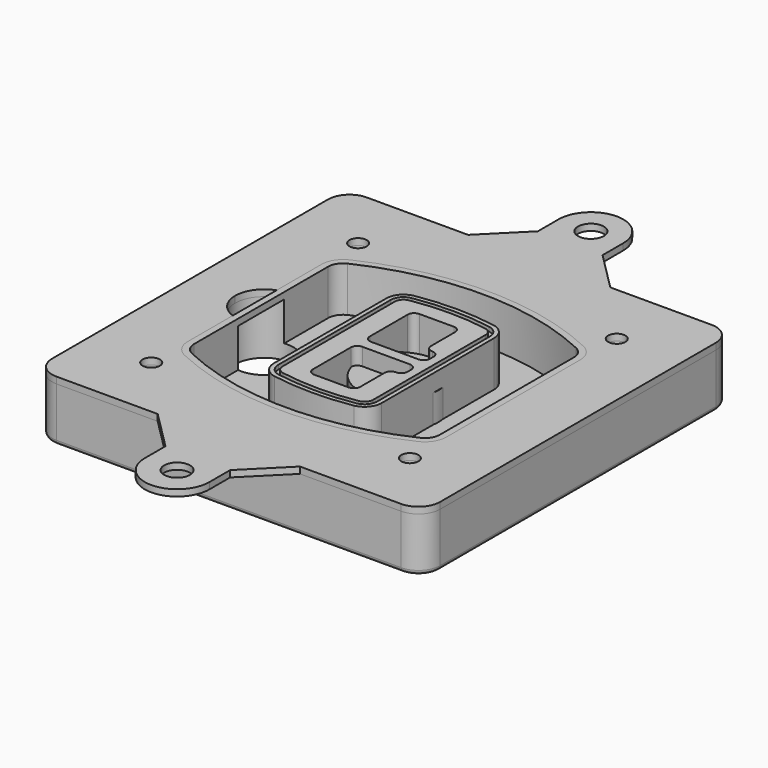
from build123d import *

# Parameters (mm, degrees)
F0_R      = 4
F1_DEPTH  = 25
F2_DEPTH  = 3
F3_DEPTH  = 18
F5_DEPTH  = 21
F6_DEPTH  = 2
F8_DEPTH  = 20
F9_DEPTH  = 16
F10_DEPTH = 25
F7_R      = 6
F7_R_2    = 4
F11_DEPTH = 6
F13_DEPTH = 9
F15_R     = 2
F16_R     = 6
F16_R_2   = 4
F17_DEPTH = 3


# Not quite as in the source:
# - a feature of the source that left no trace in its solid (it failed there, or was rolled back) is left out
# - a feature names something its author has since deleted; it is built from what else it names


with BuildPart() as f1:
    # F0 (on Top) → F1 (new body)
    with BuildSketch(Plane.XY):
        with BuildLine():
            ThreePointArc((-90, -80), (-87.0710678119, -87.0710678119), (-80, -90))
            Line((-80, -90), (80, -90))
            ThreePointArc((80, -90), (87.0710678119, -87.0710678119), (90, -80))
            Line((90, -80), (90, 80))
            ThreePointArc((90, 80), (87.0710678119, 87.0710678119), (80, 90))
            Line((80, 90), (-80, 90))
            ThreePointArc((-80, 90), (-87.0710678119, 87.0710678119), (-90, 80))
            Line((-90, 80), (-90, -80))
        make_face()
        with Locations((-60, -60)):
            Circle(F0_R, mode=Mode.SUBTRACT)
        with Locations((60, -60)):
            Circle(F0_R, mode=Mode.SUBTRACT)
        with Locations((-60, 60)):
            Circle(F0_R, mode=Mode.SUBTRACT)
        with BuildLine():
            ThreePointArc((-64, 38.8308515907), (-61.8195654598, 46.3340424013), (-55.9574468085, 51.5000594398))
            ThreePointArc((-55.9574468085, 51.5000594398), (0, 64), (55.9574468085, 51.5000594398))
            ThreePointArc((55.9574468085, 51.5000594398), (61.8195654598, 46.3340424013), (64, 38.8308515907))
            Line((64, 38.8308515907), (64, -38.8308515907))
            ThreePointArc((64, -38.8308515907), (61.8195654598, -46.3340424013), (55.9574468085, -51.5000594398))
            ThreePointArc((55.9574468085, -51.5000594398), (0, -64), (-55.9574468085, -51.5000594398))
            ThreePointArc((-55.9574468085, -51.5000594398), (-61.8195654598, -46.3340424013), (-64, -38.8308515907))
            Line((-64, -38.8308515907), (-64, 38.8308515907))
        make_face(mode=Mode.SUBTRACT)
        with Locations((60, 60)):
            Circle(F0_R, mode=Mode.SUBTRACT)
        with BuildLine():
            ThreePointArc((55.9574468085, 51.5000594398), (0, 64), (-55.9574468085, 51.5000594398))
            ThreePointArc((-55.9574468085, 51.5000594398), (-61.8195654598, 46.3340424013), (-64, 38.8308515907))
            Line((-64, 38.8308515907), (-64, -38.8308515907))
            ThreePointArc((-64, -38.8308515907), (-61.8195654598, -46.3340424013), (-55.9574468085, -51.5000594398))
            ThreePointArc((-55.9574468085, -51.5000594398), (0, -64), (55.9574468085, -51.5000594398))
            ThreePointArc((55.9574468085, -51.5000594398), (61.8195654598, -46.3340424013), (64, -38.8308515907))
            Line((64, -38.8308515907), (64, 38.8308515907))
            ThreePointArc((64, 38.8308515907), (61.8195654598, 46.3340424013), (55.9574468085, 51.5000594398))
        make_face()
        with BuildLine():
            Line((-60, -38.8308515907), (-60, 38.8308515907))
            ThreePointArc((-60, 38.8308515907), (-58.442546757, 44.1902735983), (-54.2553191489, 47.8802857686))
            ThreePointArc((-54.2553191489, 47.8802857686), (0, 60), (54.2553191489, 47.8802857686))
            ThreePointArc((54.2553191489, 47.8802857686), (58.442546757, 44.1902735983), (60, 38.8308515907))
            Line((60, 38.8308515907), (60, -38.8308515907))
            ThreePointArc((60, -38.8308515907), (58.442546757, -44.1902735983), (54.2553191489, -47.8802857686))
            ThreePointArc((54.2553191489, -47.8802857686), (0, -60), (-54.2553191489, -47.8802857686))
            ThreePointArc((-54.2553191489, -47.8802857686), (-58.442546757, -44.1902735983), (-60, -38.8308515907))
        make_face(mode=Mode.SUBTRACT)
        with BuildLine():
            ThreePointArc((-54.2553191489, 47.8802857686), (-58.442546757, 44.1902735983), (-60, 38.8308515907))
            Line((-60, 38.8308515907), (-60, -38.8308515907))
            ThreePointArc((-60, -38.8308515907), (-58.442546757, -44.1902735983), (-54.2553191489, -47.8802857686))
            ThreePointArc((-54.2553191489, -47.8802857686), (0, -60), (54.2553191489, -47.8802857686))
            ThreePointArc((54.2553191489, -47.8802857686), (58.442546757, -44.1902735983), (60, -38.8308515907))
            Line((60, -38.8308515907), (60, 38.8308515907))
            ThreePointArc((60, 38.8308515907), (58.442546757, 44.1902735983), (54.2553191489, 47.8802857686))
            ThreePointArc((54.2553191489, 47.8802857686), (0, 60), (-54.2553191489, 47.8802857686))
        make_face()
        with BuildLine():
            ThreePointArc((52.9787234043, 45.1654555152), (55.9097827299, 42.582446996), (57, 38.8308515907))
            Line((57, 38.8308515907), (57, -38.8308515907))
            ThreePointArc((57, -38.8308515907), (55.9097827299, -42.582446996), (52.9787234043, -45.1654555152))
            ThreePointArc((52.9787234043, -45.1654555152), (0, -57), (-52.9787234043, -45.1654555152))
            ThreePointArc((-52.9787234043, -45.1654555152), (-55.9097827299, -42.582446996), (-57, -38.8308515907))
            Line((-57, -38.8308515907), (-57, 38.8308515907))
            ThreePointArc((-57, 38.8308515907), (-55.9097827299, 42.582446996), (-52.9787234043, 45.1654555152))
            ThreePointArc((-52.9787234043, 45.1654555152), (0, 57), (52.9787234043, 45.1654555152))
        make_face(mode=Mode.SUBTRACT)
        with BuildLine():
            Line((57, -38.8308515907), (57, 38.8308515907))
            ThreePointArc((57, 38.8308515907), (55.9097827299, 42.582446996), (52.9787234043, 45.1654555152))
            ThreePointArc((52.9787234043, 45.1654555152), (0, 57), (-52.9787234043, 45.1654555152))
            ThreePointArc((-52.9787234043, 45.1654555152), (-55.9097827299, 42.582446996), (-57, 38.8308515907))
            Line((-57, 38.8308515907), (-57, -38.8308515907))
            ThreePointArc((-57, -38.8308515907), (-55.9097827299, -42.582446996), (-52.9787234043, -45.1654555152))
            ThreePointArc((-52.9787234043, -45.1654555152), (0, -57), (52.9787234043, -45.1654555152))
            ThreePointArc((52.9787234043, -45.1654555152), (55.9097827299, -42.582446996), (57, -38.8308515907))
        make_face()
    extrude(amount=-F1_DEPTH)

    # F0 (on Top) → F2 (join)
    with BuildSketch(Plane.XY):
        with BuildLine():
            ThreePointArc((-54.2553191489, 47.8802857686), (-58.442546757, 44.1902735983), (-60, 38.8308515907))
            Line((-60, 38.8308515907), (-60, -38.8308515907))
            ThreePointArc((-60, -38.8308515907), (-58.442546757, -44.1902735983), (-54.2553191489, -47.8802857686))
            ThreePointArc((-54.2553191489, -47.8802857686), (0, -60), (54.2553191489, -47.8802857686))
            ThreePointArc((54.2553191489, -47.8802857686), (58.442546757, -44.1902735983), (60, -38.8308515907))
            Line((60, -38.8308515907), (60, 38.8308515907))
            ThreePointArc((60, 38.8308515907), (58.442546757, 44.1902735983), (54.2553191489, 47.8802857686))
            ThreePointArc((54.2553191489, 47.8802857686), (0, 60), (-54.2553191489, 47.8802857686))
        make_face()
        with BuildLine():
            ThreePointArc((52.9787234043, 45.1654555152), (55.9097827299, 42.582446996), (57, 38.8308515907))
            Line((57, 38.8308515907), (57, -38.8308515907))
            ThreePointArc((57, -38.8308515907), (55.9097827299, -42.582446996), (52.9787234043, -45.1654555152))
            ThreePointArc((52.9787234043, -45.1654555152), (0, -57), (-52.9787234043, -45.1654555152))
            ThreePointArc((-52.9787234043, -45.1654555152), (-55.9097827299, -42.582446996), (-57, -38.8308515907))
            Line((-57, -38.8308515907), (-57, 38.8308515907))
            ThreePointArc((-57, 38.8308515907), (-55.9097827299, 42.582446996), (-52.9787234043, 45.1654555152))
            ThreePointArc((-52.9787234043, 45.1654555152), (0, 57), (52.9787234043, 45.1654555152))
        make_face(mode=Mode.SUBTRACT)
    extrude(amount=F2_DEPTH)

    # F0 (on Top) → F3 (cut)
    with BuildSketch(Plane.XY):
        with BuildLine():
            Line((57, -38.8308515907), (57, 38.8308515907))
            ThreePointArc((57, 38.8308515907), (55.9097827299, 42.582446996), (52.9787234043, 45.1654555152))
            ThreePointArc((52.9787234043, 45.1654555152), (0, 57), (-52.9787234043, 45.1654555152))
            ThreePointArc((-52.9787234043, 45.1654555152), (-55.9097827299, 42.582446996), (-57, 38.8308515907))
            Line((-57, 38.8308515907), (-57, -38.8308515907))
            ThreePointArc((-57, -38.8308515907), (-55.9097827299, -42.582446996), (-52.9787234043, -45.1654555152))
            ThreePointArc((-52.9787234043, -45.1654555152), (0, -57), (52.9787234043, -45.1654555152))
            ThreePointArc((52.9787234043, -45.1654555152), (55.9097827299, -42.582446996), (57, -38.8308515907))
        make_face()
    extrude(amount=-F3_DEPTH, mode=Mode.SUBTRACT)

    # F4 (on face) → F5 (join, through all)
    with BuildSketch(Plane.XY.offset(3)):
        with BuildLine():
            ThreePointArc((-25, -32.5662280692), (-23.1122504785, -37.7276614059), (-18.3399014778, -40.4532214146))
            ThreePointArc((-18.3399014778, -40.4532214146), (0, -42), (18.3399014778, -40.4532214146))
            ThreePointArc((18.3399014778, -40.4532214146), (23.1122504785, -37.7276614059), (25, -32.5662280692))
            Line((25, -32.5662280692), (25, 32.5662280692))
            ThreePointArc((25, 32.5662280692), (23.1122504785, 37.7276614059), (18.3399014778, 40.4532214146))
            ThreePointArc((18.3399014778, 40.4532214146), (0, 42), (-18.3399014778, 40.4532214146))
            ThreePointArc((-18.3399014778, 40.4532214146), (-23.1122504785, 37.7276614059), (-25, 32.5662280692))
            Line((-25, 32.5662280692), (-25, -32.5662280692))
        make_face()
        with BuildLine():
            ThreePointArc((18.0049261084, 38.4814730782), (21.5841878588, 36.4373030717), (23, 32.5662280692))
            Line((23, 32.5662280692), (23, -32.5662280692))
            ThreePointArc((23, -32.5662280692), (21.5841878588, -36.4373030717), (18.0049261084, -38.4814730782))
            ThreePointArc((18.0049261084, -38.4814730782), (0, -40), (-18.0049261084, -38.4814730782))
            ThreePointArc((-18.0049261084, -38.4814730782), (-21.5841878588, -36.4373030717), (-23, -32.5662280692))
            Line((-23, -32.5662280692), (-23, 32.5662280692))
            ThreePointArc((-23, 32.5662280692), (-21.5841878588, 36.4373030717), (-18.0049261084, 38.4814730782))
            ThreePointArc((-18.0049261084, 38.4814730782), (0, 40), (18.0049261084, 38.4814730782))
        make_face(mode=Mode.SUBTRACT)
        with BuildLine():
            Line((23, -32.5662280692), (23, 32.5662280692))
            ThreePointArc((23, 32.5662280692), (21.5841878588, 36.4373030717), (18.0049261084, 38.4814730782))
            ThreePointArc((18.0049261084, 38.4814730782), (0, 40), (-18.0049261084, 38.4814730782))
            ThreePointArc((-18.0049261084, 38.4814730782), (-21.5841878588, 36.4373030717), (-23, 32.5662280692))
            Line((-23, 32.5662280692), (-23, -32.5662280692))
            ThreePointArc((-23, -32.5662280692), (-21.5841878588, -36.4373030717), (-18.0049261084, -38.4814730782))
            ThreePointArc((-18.0049261084, -38.4814730782), (0, -40), (18.0049261084, -38.4814730782))
            ThreePointArc((18.0049261084, -38.4814730782), (21.5841878588, -36.4373030717), (23, -32.5662280692))
        make_face()
        with BuildLine():
            ThreePointArc((17.6699507389, 36.5097247419), (20.0561252392, 35.1469447375), (21, 32.5662280692))
            Line((21, 32.5662280692), (21, -32.5662280692))
            ThreePointArc((21, -32.5662280692), (20.0561252392, -35.1469447375), (17.6699507389, -36.5097247419))
            ThreePointArc((17.6699507389, -36.5097247419), (0, -38), (-17.6699507389, -36.5097247419))
            ThreePointArc((-17.6699507389, -36.5097247419), (-20.0561252392, -35.1469447375), (-21, -32.5662280692))
            Line((-21, -32.5662280692), (-21, 32.5662280692))
            ThreePointArc((-21, 32.5662280692), (-20.0561252392, 35.1469447375), (-17.6699507389, 36.5097247419))
            ThreePointArc((-17.6699507389, 36.5097247419), (0, 38), (17.6699507389, 36.5097247419))
        make_face(mode=Mode.SUBTRACT)
        with BuildLine():
            Line((21, -32.5662280692), (21, 32.5662280692))
            ThreePointArc((21, 32.5662280692), (20.0561252392, 35.1469447375), (17.6699507389, 36.5097247419))
            ThreePointArc((17.6699507389, 36.5097247419), (0, 38), (-17.6699507389, 36.5097247419))
            ThreePointArc((-17.6699507389, 36.5097247419), (-20.0561252392, 35.1469447375), (-21, 32.5662280692))
            Line((-21, 32.5662280692), (-21, -32.5662280692))
            ThreePointArc((-21, -32.5662280692), (-20.0561252392, -35.1469447375), (-17.6699507389, -36.5097247419))
            ThreePointArc((-17.6699507389, -36.5097247419), (0, -38), (17.6699507389, -36.5097247419))
            ThreePointArc((17.6699507389, -36.5097247419), (20.0561252392, -35.1469447375), (21, -32.5662280692))
        make_face()
        with BuildLine():
            Line((-8, -2.5), (14, -2.5))
            ThreePointArc((14, -2.5), (16.1213203436, -3.3786796564), (17, -5.5))
            Line((17, -5.5), (17, -7.5))
            ThreePointArc((17, -7.5), (16.1213203436, -9.6213203436), (14, -10.5))
            ThreePointArc((14, -10.5), (11.8786796564, -11.3786796564), (11, -13.5))
            Line((11, -13.5), (11, -27.5))
            ThreePointArc((11, -27.5), (10.1213203436, -29.6213203436), (8, -30.5))
            Line((8, -30.5), (-8, -30.5))
            ThreePointArc((-8, -30.5), (-10.1213203436, -29.6213203436), (-11, -27.5))
            Line((-11, -27.5), (-11, -5.5))
            ThreePointArc((-11, -5.5), (-10.1213203436, -3.3786796564), (-8, -2.5))
        make_face(mode=Mode.SUBTRACT)
        with BuildLine():
            ThreePointArc((-8, 2.5), (-10.1213203436, 3.3786796564), (-11, 5.5))
            Line((-11, 5.5), (-11, 27.5))
            ThreePointArc((-11, 27.5), (-10.1213203436, 29.6213203436), (-8, 30.5))
            Line((-8, 30.5), (8, 30.5))
            ThreePointArc((8, 30.5), (10.1213203436, 29.6213203436), (11, 27.5))
            Line((11, 27.5), (11, 13.5))
            ThreePointArc((11, 13.5), (11.8786796564, 11.3786796564), (14, 10.5))
            ThreePointArc((14, 10.5), (16.1213203436, 9.6213203436), (17, 7.5))
            Line((17, 7.5), (17, 5.5))
            ThreePointArc((17, 5.5), (16.1213203436, 3.3786796564), (14, 2.5))
            Line((14, 2.5), (-8, 2.5))
        make_face(mode=Mode.SUBTRACT)
    extrude(amount=-F5_DEPTH)

    # F4 (on face) → F6 (cut)
    with BuildSketch(Plane.XY.offset(3)):
        with BuildLine():
            Line((23, -32.5662280692), (23, 32.5662280692))
            ThreePointArc((23, 32.5662280692), (21.5841878588, 36.4373030717), (18.0049261084, 38.4814730782))
            ThreePointArc((18.0049261084, 38.4814730782), (0, 40), (-18.0049261084, 38.4814730782))
            ThreePointArc((-18.0049261084, 38.4814730782), (-21.5841878588, 36.4373030717), (-23, 32.5662280692))
            Line((-23, 32.5662280692), (-23, -32.5662280692))
            ThreePointArc((-23, -32.5662280692), (-21.5841878588, -36.4373030717), (-18.0049261084, -38.4814730782))
            ThreePointArc((-18.0049261084, -38.4814730782), (0, -40), (18.0049261084, -38.4814730782))
            ThreePointArc((18.0049261084, -38.4814730782), (21.5841878588, -36.4373030717), (23, -32.5662280692))
        make_face()
        with BuildLine():
            ThreePointArc((17.6699507389, 36.5097247419), (20.0561252392, 35.1469447375), (21, 32.5662280692))
            Line((21, 32.5662280692), (21, -32.5662280692))
            ThreePointArc((21, -32.5662280692), (20.0561252392, -35.1469447375), (17.6699507389, -36.5097247419))
            ThreePointArc((17.6699507389, -36.5097247419), (0, -38), (-17.6699507389, -36.5097247419))
            ThreePointArc((-17.6699507389, -36.5097247419), (-20.0561252392, -35.1469447375), (-21, -32.5662280692))
            Line((-21, -32.5662280692), (-21, 32.5662280692))
            ThreePointArc((-21, 32.5662280692), (-20.0561252392, 35.1469447375), (-17.6699507389, 36.5097247419))
            ThreePointArc((-17.6699507389, 36.5097247419), (0, 38), (17.6699507389, 36.5097247419))
        make_face(mode=Mode.SUBTRACT)
    extrude(amount=-F6_DEPTH, mode=Mode.SUBTRACT)

    # F7 (on face) → F8 (join)
    with BuildSketch(Plane(origin=(0, 0, -25), x_dir=(1, 0, 0), z_dir=(0, 0, -1))):
        with BuildLine():
            ThreePointArc((-6.71157564, 0), (6.7567035675, 13.4682792075), (20.224982775, 0))
            Line((20.224982775, 0), (25.224982775, 0))
            ThreePointArc((25.224982775, 0), (6.7567035675, 18.4682792075), (-11.71157564, 0))
            Line((-11.71157564, 0), (-6.71157564, 0))
        make_face()
        with BuildLine():
            Line((-6.71157564, 0), (20.224982775, 0))
            ThreePointArc((20.224982775, 0), (6.7567035675, 13.4682792075), (-6.71157564, 0))
        make_face()
        with BuildLine():
            ThreePointArc((-6.71157564, 0), (6.7567035675, -13.4682792075), (20.224982775, 0))
            Line((20.224982775, 0), (-6.71157564, 0))
        make_face()
        with BuildLine():
            Line((25.224982775, 0), (20.224982775, 0))
            ThreePointArc((20.224982775, 0), (6.7567035675, -13.4682792075), (-6.71157564, 0))
            Line((-6.71157564, 0), (-11.71157564, 0))
            ThreePointArc((-11.71157564, 0), (6.7567035675, -18.4682792075), (25.224982775, 0))
        make_face()
    extrude(amount=-F8_DEPTH)

    # F7 (on face) → F9 (cut)
    with BuildSketch(Plane(origin=(0, 0, -25), x_dir=(1, 0, 0), z_dir=(0, 0, -1))):
        with BuildLine():
            Line((-6.71157564, 0), (20.224982775, 0))
            ThreePointArc((20.224982775, 0), (6.7567035675, 13.4682792075), (-6.71157564, 0))
        make_face()
        with BuildLine():
            ThreePointArc((-6.71157564, 0), (6.7567035675, -13.4682792075), (20.224982775, 0))
            Line((20.224982775, 0), (-6.71157564, 0))
        make_face()
    extrude(amount=-F9_DEPTH, mode=Mode.SUBTRACT)

    # F7 (on face) → F10 (cut)
    with BuildSketch(Plane(origin=(0, 0, -25), x_dir=(1, 0, 0), z_dir=(0, 0, -1))):
        with BuildLine():
            Line((-69.0318229325, 0), (-42.0952645175, 0))
            ThreePointArc((-42.0952645175, 0), (-55.563543725, 13.4682792075), (-69.0318229325, 0))
        make_face()
        with BuildLine():
            ThreePointArc((-69.0318229325, 0), (-55.563543725, -13.4682792075), (-42.0952645175, 0))
            Line((-42.0952645175, 0), (-69.0318229325, 0))
        make_face()
    extrude(amount=-F10_DEPTH, mode=Mode.SUBTRACT)

    # F7 (on face) → F11 (cut)
    with BuildSketch(Plane(origin=(0, 0, -25), x_dir=(1, 0, 0), z_dir=(0, 0, -1))):
        with Locations((60, -60)):
            Circle(F7_R)
        with Locations((60, -60)):
            Circle(F7_R_2, mode=Mode.SUBTRACT)
        with Locations((-60, -60)):
            Circle(F7_R)
        with Locations((-60, -60)):
            Circle(F7_R_2, mode=Mode.SUBTRACT)
        with Locations((-60, 60)):
            Circle(F7_R)
        with Locations((-60, 60)):
            Circle(F7_R_2, mode=Mode.SUBTRACT)
        with Locations((60, 60)):
            Circle(F7_R)
        with Locations((60, 60)):
            Circle(F7_R_2, mode=Mode.SUBTRACT)
    extrude(amount=-F11_DEPTH, mode=Mode.SUBTRACT)

    # F12 (on face) → F13 (cut, through all)
    with BuildSketch(Plane(origin=(0, 0, -9), x_dir=(1, 0, 0), z_dir=(0, 0, -1))):
        with BuildLine():
            ThreePointArc((20.224982775, 0), (20.1663399806, 1.2554664788), (19.9909222755, 2.5))
            Line((19.9909222755, 2.5), (14, 2.5))
            ThreePointArc((14, 2.5), (16.1213203436, 3.3786796564), (17, 5.5))
            Line((17, 5.5), (17, 7.5))
            ThreePointArc((17, 7.5), (16.1213203436, 9.6213203436), (14, 10.5))
            ThreePointArc((14, 10.5), (12.1627255951, 11.1284134507), (11.0951631559, 12.750384826))
            ThreePointArc((11.0951631559, 12.750384826), (11.0476113807, 12.7664660322), (11, 12.7823698976))
            Line((11, 12.7823698976), (11, -12.7823698976))
            ThreePointArc((11, -12.7823698976), (11.0476113807, -12.7664660322), (11.0951631559, -12.750384826))
            ThreePointArc((11.0951631559, -12.750384826), (12.1627255951, -11.1284134507), (14, -10.5))
            ThreePointArc((14, -10.5), (16.1213203436, -9.6213203436), (17, -7.5))
            Line((17, -7.5), (17, -5.5))
            ThreePointArc((17, -5.5), (16.1213203436, -3.3786796564), (14, -2.5))
            Line((14, -2.5), (19.9909222755, -2.5))
            ThreePointArc((19.9909222755, -2.5), (20.1663399806, -1.2554664788), (20.224982775, 0))
        make_face()
    extrude(amount=F13_DEPTH, mode=Mode.SUBTRACT)

    # F15
    f15_edges = [f1.edges().sort_by_distance(p)[0] for p in [
        (0, -90, -25),
        (-87.071068, -87.071068, -25),
        (-90, 0, -25),
        (-87.071068, 87.071068, -25),
        (87.071068, -87.071068, -25),
        (0, 90, -25),
        (90, 0, -25),
        (87.071068, 87.071068, -25),
    ]]
    fillet(f15_edges, radius=F15_R)


with BuildPart() as f17:
    # F16 (on face) → F17 (new body, through all)
    with BuildSketch(Plane.XY):
        with BuildLine():
            Line((-15, 108), (-33, 90))
            Line((-33, 90), (33, 90))
            Line((33, 90), (15, 108))
            Line((15, 108), (15, 120))
            ThreePointArc((15, 120), (0, 135), (-15, 120))
            Line((-15, 120), (-15, 108))
        make_face()
        with Locations((0, 120)):
            Circle(F16_R, mode=Mode.SUBTRACT)
        with BuildLine():
            Line((-33, 90), (-80, 90))
            ThreePointArc((-80, 90), (-87.0710678119, 87.0710678119), (-90, 80))
            Line((-90, 80), (-90, -80))
            ThreePointArc((-90, -80), (-87.0710678119, -87.0710678119), (-80, -90))
            Line((-80, -90), (-33, -90))
            Line((-33, -90), (33, -90))
            Line((33, -90), (80, -90))
            ThreePointArc((80, -90), (87.0710678119, -87.0710678119), (90, -80))
            Line((90, -80), (90, 80))
            ThreePointArc((90, 80), (87.0710678119, 87.0710678119), (80, 90))
            Line((80, 90), (33, 90))
            Line((33, 90), (-33, 90))
        make_face()
        with Locations((-60, -60)):
            Circle(F16_R_2, mode=Mode.SUBTRACT)
        with Locations((60, -60)):
            Circle(F16_R_2, mode=Mode.SUBTRACT)
        with Locations((-60, 60)):
            Circle(F16_R_2, mode=Mode.SUBTRACT)
        with BuildLine():
            ThreePointArc((-60, 38.8308515907), (-58.442546757, 44.1902735983), (-54.2553191489, 47.8802857686))
            ThreePointArc((-54.2553191489, 47.8802857686), (0, 60), (54.2553191489, 47.8802857686))
            ThreePointArc((54.2553191489, 47.8802857686), (58.442546757, 44.1902735983), (60, 38.8308515907))
            Line((60, 38.8308515907), (60, -38.8308515907))
            ThreePointArc((60, -38.8308515907), (58.442546757, -44.1902735983), (54.2553191489, -47.8802857686))
            ThreePointArc((54.2553191489, -47.8802857686), (0, -60), (-54.2553191489, -47.8802857686))
            ThreePointArc((-54.2553191489, -47.8802857686), (-58.442546757, -44.1902735983), (-60, -38.8308515907))
            Line((-60, -38.8308515907), (-60, -12.7166190685))
            ThreePointArc((-60, -12.7166190685), (-66.5441169481, -7.798817635), (-69.0318229325, 0))
            ThreePointArc((-69.0318229325, 0), (-66.5441169481, 7.798817635), (-60, 12.7166190685))
            Line((-60, 12.7166190685), (-60, 38.8308515907))
        make_face(mode=Mode.SUBTRACT)
        with Locations((60, 60)):
            Circle(F16_R_2, mode=Mode.SUBTRACT)
        with BuildLine():
            Line((33, -90), (-33, -90))
            Line((-33, -90), (-15, -108))
            Line((-15, -108), (-15, -120))
            ThreePointArc((-15, -120), (0, -135), (15, -120))
            Line((15, -120), (15, -108))
            Line((15, -108), (33, -90))
        make_face()
        with Locations((0, -120)):
            Circle(F16_R, mode=Mode.SUBTRACT)
    extrude(amount=F17_DEPTH)


solid = Compound([f1.part, f17.part])
